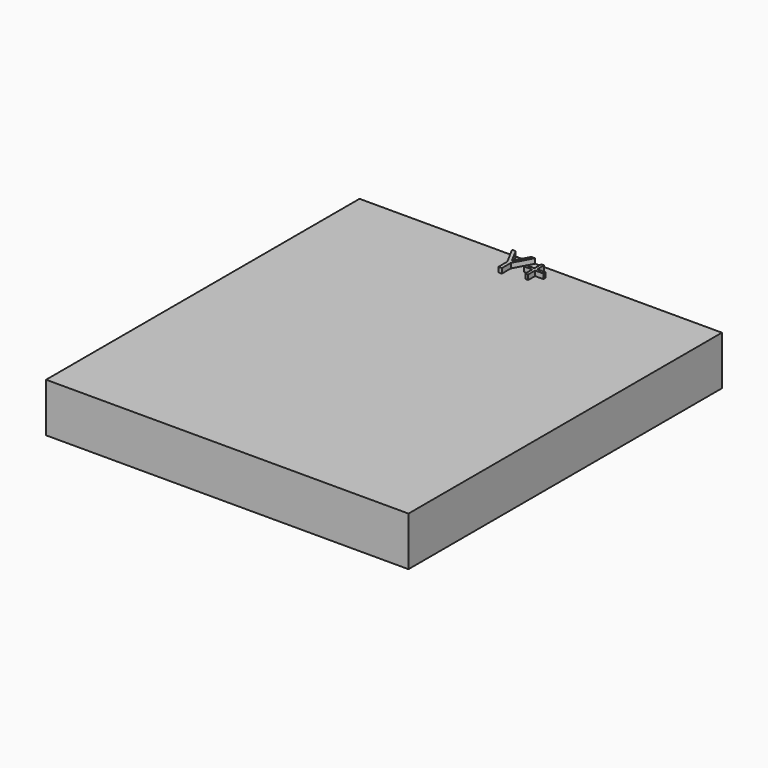
from build123d import *

# Parameters (mm, degrees)
F0_W         = 20
F0_H         = 20
F1_DEPTH     = 25
F2_W         = 148
F2_H         = 160
F3_DEPTH     = 20
F4_TEXT_SIZE = 16.7248358743
F5_DEPTH     = 2


# Not quite as in the source:
# - Text() gives the source's letters only with a copy of the font that has no kerning and outlines rounded to 1/6400 em; it was checked with that copy


with BuildPart() as f1:
    # F0 (on Top) → F1 (new body)
    with BuildSketch(Plane.XY):
        with Locations((5.7402232289, -3.0745358765)):
            Rectangle(F0_W, F0_H)
    extrude(amount=F1_DEPTH)

    # F2 (on face) → F3 (join)
    with BuildSketch(Plane.XY.offset(25)):
        with Locations((5.7402232289, -3.0745358765)):
            Rectangle(F2_W, F2_H)
    extrude(amount=F3_DEPTH)

    # F4 (on face) → F5 (join)
    with BuildSketch(Plane.XY.offset(45)):
        with Locations((-5.9012309648, 64.883582294)):
            Text('Y+', F4_TEXT_SIZE, font='Open Sans', text_align=(TextAlign.LEFT, TextAlign.BOTTOM))
    extrude(amount=F5_DEPTH)


solid = f1.part
